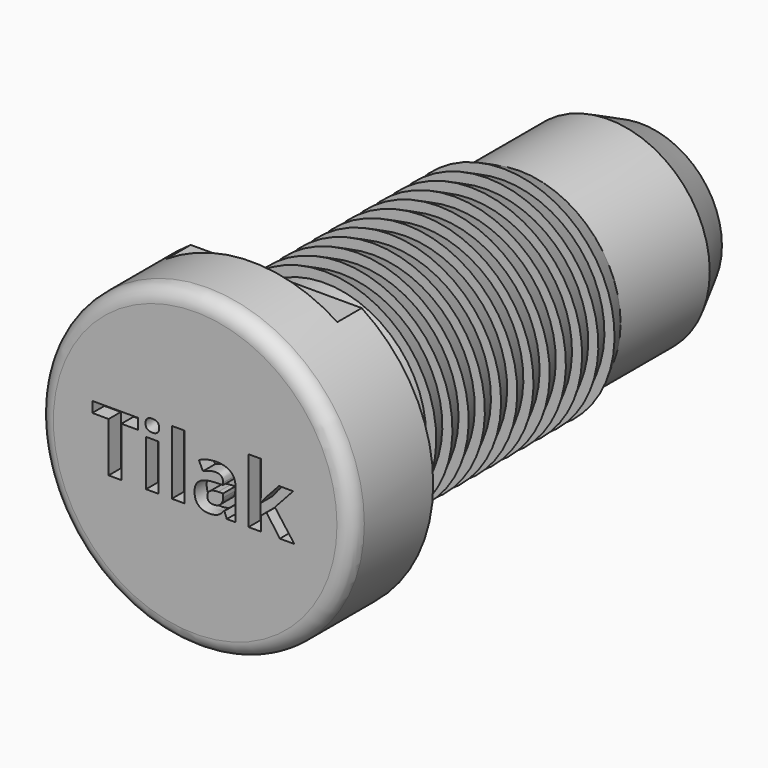
from build123d import *

# Parameters (mm, degrees)
F0_R          = 10
F1_DEPTH      = 45
F2_R          = 15.5
F3_DEPTH      = 10
F5_DEPTH      = 3
F8_SIZE2      = 2
F8_SIZE       = 4
F9_R          = 1.5
F10_TEXT_SIZE = 8.3333333333
F11_DEPTH     = 1.5


# Not quite as in the source:
# - Text() gives the source's letters only with a copy of the font that has no kerning and outlines rounded to 1/6400 em; it was checked with that copy


with BuildPart() as f1:
    # F0 (on Front) → F1 (new body)
    with BuildSketch(Plane.XZ):
        Circle(F0_R)
    extrude(amount=-F1_DEPTH)

    # F2 (on face) → F3 (join)
    with BuildSketch(Plane.XZ):
        Circle(F2_R)
    extrude(amount=F3_DEPTH)

    # F4 (on face) → F5 (cut)
    with BuildSketch(Plane(origin=(0, 0, 0), x_dir=(-1, 0, 0), z_dir=(0, 1, 0))):
        with BuildLine():
            ThreePointArc((8.4409715081, 13), (0, 15.5), (-8.4409715081, 13))
            Line((-8.4409715081, 13), (8.4409715081, 13))
        make_face()
    extrude(amount=-F5_DEPTH, mode=Mode.SUBTRACT)

    # F6 (on Right) → F7 (revolve)
    with BuildSketch(Plane.YZ):
        Polygon((28, 10), (30, 10), (28, 11), align=None)
        Polygon((6, 10), (8, 10), (6, 11), align=None)
        Polygon((8, 10), (10, 10), (8, 11), align=None)
        Polygon((10, 10), (12, 10), (10, 11), align=None)
        Polygon((12, 10), (14, 10), (12, 11), align=None)
        Polygon((14, 10), (16, 10), (14, 11), align=None)
        Polygon((16, 10), (18, 10), (16, 11), align=None)
        Polygon((18, 10), (20, 10), (18, 11), align=None)
        Polygon((20, 10), (22, 10), (20, 11), align=None)
        Polygon((22, 10), (24, 10), (22, 11), align=None)
        Polygon((24, 10), (26, 10), (24, 11), align=None)
        Polygon((26, 10), (28, 10), (26, 11), align=None)
    revolve(axis=Axis((0, 13.405341655, 0), (0, -1, 0)))

    # F8
    f8_edges = [f1.edges().sort_by_distance(p)[0] for p in [
        (-10, 45, 0),
    ]]
    chamfer(f8_edges, length=F8_SIZE, length2=F8_SIZE2)

    # F9
    f9_edges = [f1.edges().sort_by_distance(p)[0] for p in [
        (-10, 0, 0),
        (-15.5, -10, 0),
    ]]
    fillet(f9_edges, radius=F9_R)

    # F10 (on face) → F11 (cut)
    with BuildSketch(Plane.XZ.offset(10)):
        with Locations((-10.3268229167, -3)):
            Text('Tilak', F10_TEXT_SIZE, font='Open Sans', font_style=FontStyle.BOLD, text_align=(TextAlign.LEFT, TextAlign.BOTTOM))
    extrude(amount=-F11_DEPTH, mode=Mode.SUBTRACT)


solid = f1.part
